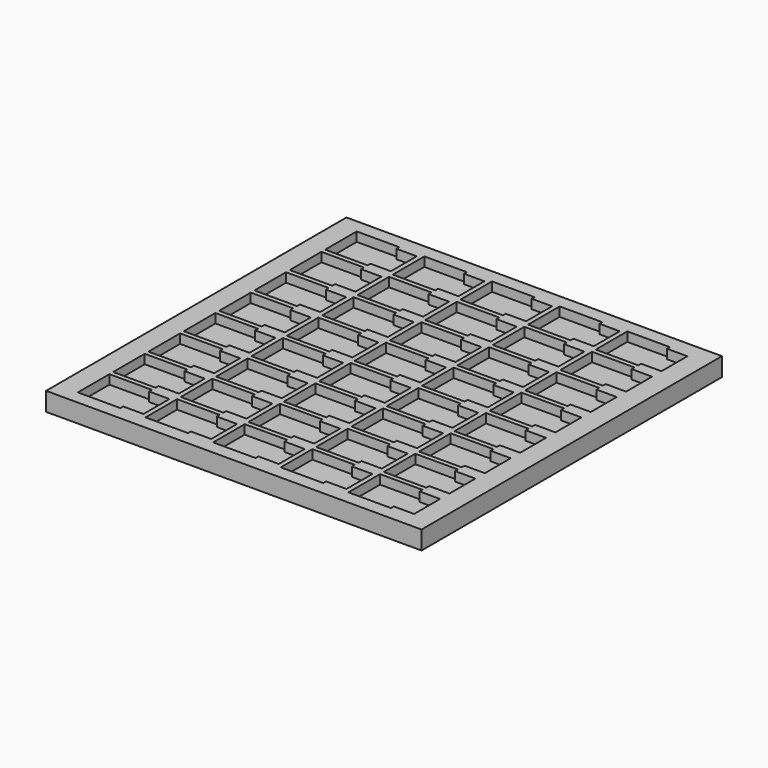
from build123d import *

# Parameters (mm, degrees)
F0_W     = 101.5
F0_H     = 101.5
F1_DEPTH = 5
F2_DEPTH = 2.5


# Not quite as in the source:
# - a feature names something its author has since deleted; it is built from what else it names


with BuildPart() as f1:
    # F0 (on Top) → F1 (new body)
    with BuildSketch(Plane.XY):
        Rectangle(F0_W, F0_H)
        Polygon((-33.5731, -46.1647), (-33.5731, -47.1182), (-45.0731, -47.1182), (-45.0731, -36.4482), (-33.5731, -36.4482), (-33.5731, -37.4017), (-28.0731, -37.4017), (-28.0731, -46.1647), align=None, mode=Mode.SUBTRACT)
        Polygon((-33.5731, -34.2267), (-33.5731, -35.1802), (-45.0731, -35.1802), (-45.0731, -24.5102), (-33.5731, -24.5102), (-33.5731, -25.4637), (-28.0731, -25.4637), (-28.0731, -34.2267), align=None, mode=Mode.SUBTRACT)
        Polygon((-15.2851, -46.1647), (-15.2851, -47.1182), (-26.7851, -47.1182), (-26.7851, -36.4482), (-15.2851, -36.4482), (-15.2851, -37.4017), (-9.7851, -37.4017), (-9.7851, -46.1647), align=None, mode=Mode.SUBTRACT)
        Polygon((-15.2851, -34.2267), (-15.2851, -35.1802), (-26.7851, -35.1802), (-26.7851, -24.5102), (-15.2851, -24.5102), (-15.2851, -25.4637), (-9.7851, -25.4637), (-9.7851, -34.2267), align=None, mode=Mode.SUBTRACT)
        Polygon((-33.5731, -22.2887), (-33.5731, -23.2422), (-45.0731, -23.2422), (-45.0731, -12.5722), (-33.5731, -12.5722), (-33.5731, -13.5257), (-28.0731, -13.5257), (-28.0731, -22.2887), align=None, mode=Mode.SUBTRACT)
        Polygon((-33.5731, -10.3507), (-33.5731, -11.3042), (-45.0731, -11.3042), (-45.0731, -0.6342), (-33.5731, -0.6342), (-33.5731, -1.5877), (-28.0731, -1.5877), (-28.0731, -10.3507), align=None, mode=Mode.SUBTRACT)
        Polygon((-15.2851, -22.2887), (-15.2851, -23.2422), (-26.7851, -23.2422), (-26.7851, -12.5722), (-15.2851, -12.5722), (-15.2851, -13.5257), (-9.7851, -13.5257), (-9.7851, -22.2887), align=None, mode=Mode.SUBTRACT)
        Polygon((-15.2851, -10.3507), (-15.2851, -11.3042), (-26.7851, -11.3042), (-26.7851, -0.6342), (-15.2851, -0.6342), (-15.2851, -1.5877), (-9.7851, -1.5877), (-9.7851, -10.3507), align=None, mode=Mode.SUBTRACT)
        Polygon((3.0029, -46.1647), (3.0029, -47.1182), (-8.4971, -47.1182), (-8.4971, -36.4482), (3.0029, -36.4482), (3.0029, -37.4017), (8.5029, -37.4017), (8.5029, -46.1647), align=None, mode=Mode.SUBTRACT)
        Polygon((21.2909, -46.1647), (21.2909, -47.1182), (9.7909, -47.1182), (9.7909, -36.4482), (21.2909, -36.4482), (21.2909, -37.4017), (26.7909, -37.4017), (26.7909, -46.1647), align=None, mode=Mode.SUBTRACT)
        Polygon((3.0029, -34.2267), (3.0029, -35.1802), (-8.4971, -35.1802), (-8.4971, -24.5102), (3.0029, -24.5102), (3.0029, -25.4637), (8.5029, -25.4637), (8.5029, -34.2267), align=None, mode=Mode.SUBTRACT)
        Polygon((21.2909, -34.2267), (21.2909, -35.1802), (9.7909, -35.1802), (9.7909, -24.5102), (21.2909, -24.5102), (21.2909, -25.4637), (26.7909, -25.4637), (26.7909, -34.2267), align=None, mode=Mode.SUBTRACT)
        Polygon((39.5789, -46.1647), (39.5789, -47.1182), (28.0789, -47.1182), (28.0789, -36.4482), (39.5789, -36.4482), (39.5789, -37.4017), (45.0789, -37.4017), (45.0789, -46.1647), align=None, mode=Mode.SUBTRACT)
        Polygon((39.5789, -34.2267), (39.5789, -35.1802), (28.0789, -35.1802), (28.0789, -24.5102), (39.5789, -24.5102), (39.5789, -25.4637), (45.0789, -25.4637), (45.0789, -34.2267), align=None, mode=Mode.SUBTRACT)
        Polygon((3.0029, -22.2887), (3.0029, -23.2422), (-8.4971, -23.2422), (-8.4971, -12.5722), (3.0029, -12.5722), (3.0029, -13.5257), (8.5029, -13.5257), (8.5029, -22.2887), align=None, mode=Mode.SUBTRACT)
        Polygon((21.2909, -22.2887), (21.2909, -23.2422), (9.7909, -23.2422), (9.7909, -12.5722), (21.2909, -12.5722), (21.2909, -13.5257), (26.7909, -13.5257), (26.7909, -22.2887), align=None, mode=Mode.SUBTRACT)
        Polygon((3.0029, -10.3507), (3.0029, -11.3042), (-8.4971, -11.3042), (-8.4971, -0.6342), (3.0029, -0.6342), (3.0029, -1.5877), (8.5029, -1.5877), (8.5029, -10.3507), align=None, mode=Mode.SUBTRACT)
        Polygon((21.2909, -10.3507), (21.2909, -11.3042), (9.7909, -11.3042), (9.7909, -0.6342), (21.2909, -0.6342), (21.2909, -1.5877), (26.7909, -1.5877), (26.7909, -10.3507), align=None, mode=Mode.SUBTRACT)
        Polygon((39.5789, -22.2887), (39.5789, -23.2422), (28.0789, -23.2422), (28.0789, -12.5722), (39.5789, -12.5722), (39.5789, -13.5257), (45.0789, -13.5257), (45.0789, -22.2887), align=None, mode=Mode.SUBTRACT)
        Polygon((39.5789, -10.3507), (39.5789, -11.3042), (28.0789, -11.3042), (28.0789, -0.6342), (39.5789, -0.6342), (39.5789, -1.5877), (45.0789, -1.5877), (45.0789, -10.3507), align=None, mode=Mode.SUBTRACT)
        Polygon((-33.5731, 1.5873), (-33.5731, 0.6338), (-45.0731, 0.6338), (-45.0731, 11.3038), (-33.5731, 11.3038), (-33.5731, 10.3503), (-28.0731, 10.3503), (-28.0731, 1.5873), align=None, mode=Mode.SUBTRACT)
        Polygon((-33.5731, 13.5253), (-33.5731, 12.5718), (-45.0731, 12.5718), (-45.0731, 23.2418), (-33.5731, 23.2418), (-33.5731, 22.2883), (-28.0731, 22.2883), (-28.0731, 13.5253), align=None, mode=Mode.SUBTRACT)
        Polygon((-15.2851, 1.5873), (-15.2851, 0.6338), (-26.7851, 0.6338), (-26.7851, 11.3038), (-15.2851, 11.3038), (-15.2851, 10.3503), (-9.7851, 10.3503), (-9.7851, 1.5873), align=None, mode=Mode.SUBTRACT)
        Polygon((-15.2851, 13.5253), (-15.2851, 12.5718), (-26.7851, 12.5718), (-26.7851, 23.2418), (-15.2851, 23.2418), (-15.2851, 22.2883), (-9.7851, 22.2883), (-9.7851, 13.5253), align=None, mode=Mode.SUBTRACT)
        Polygon((-33.5731, 25.4633), (-33.5731, 24.5098), (-45.0731, 24.5098), (-45.0731, 35.1798), (-33.5731, 35.1798), (-33.5731, 34.2263), (-28.0731, 34.2263), (-28.0731, 25.4633), align=None, mode=Mode.SUBTRACT)
        Polygon((-45.0731, 36.4478), (-45.0731, 47.1178), (-33.5731, 47.1178), (-33.5731, 46.1643), (-28.0731, 46.1643), (-28.0731, 37.4013), (-33.5731, 37.4013), (-33.5731, 36.4478), align=None, mode=Mode.SUBTRACT)
        Polygon((-15.2851, 25.4633), (-15.2851, 24.5098), (-26.7851, 24.5098), (-26.7851, 35.1798), (-15.2851, 35.1798), (-15.2851, 34.2263), (-9.7851, 34.2263), (-9.7851, 25.4633), align=None, mode=Mode.SUBTRACT)
        Polygon((-15.2851, 37.4013), (-15.2851, 36.4478), (-26.7851, 36.4478), (-26.7851, 47.1178), (-15.2851, 47.1178), (-15.2851, 46.1643), (-9.7851, 46.1643), (-9.7851, 37.4013), align=None, mode=Mode.SUBTRACT)
        Polygon((3.0029, 1.5873), (3.0029, 0.6338), (-8.4971, 0.6338), (-8.4971, 11.3038), (3.0029, 11.3038), (3.0029, 10.3503), (8.5029, 10.3503), (8.5029, 1.5873), align=None, mode=Mode.SUBTRACT)
        Polygon((21.2909, 1.5873), (21.2909, 0.6338), (9.7909, 0.6338), (9.7909, 11.3038), (21.2909, 11.3038), (21.2909, 10.3503), (26.7909, 10.3503), (26.7909, 1.5873), align=None, mode=Mode.SUBTRACT)
        Polygon((3.0029, 13.5253), (3.0029, 12.5718), (-8.4971, 12.5718), (-8.4971, 23.2418), (3.0029, 23.2418), (3.0029, 22.2883), (8.5029, 22.2883), (8.5029, 13.5253), align=None, mode=Mode.SUBTRACT)
        Polygon((21.2909, 13.5253), (21.2909, 12.5718), (9.7909, 12.5718), (9.7909, 23.2418), (21.2909, 23.2418), (21.2909, 22.2883), (26.7909, 22.2883), (26.7909, 13.5253), align=None, mode=Mode.SUBTRACT)
        Polygon((39.5789, 1.5873), (39.5789, 0.6338), (28.0789, 0.6338), (28.0789, 11.3038), (39.5789, 11.3038), (39.5789, 10.3503), (45.0789, 10.3503), (45.0789, 1.5873), align=None, mode=Mode.SUBTRACT)
        Polygon((39.5789, 13.5253), (39.5789, 12.5718), (28.0789, 12.5718), (28.0789, 23.2418), (39.5789, 23.2418), (39.5789, 22.2883), (45.0789, 22.2883), (45.0789, 13.5253), align=None, mode=Mode.SUBTRACT)
        Polygon((3.0029, 25.4633), (3.0029, 24.5098), (-8.4971, 24.5098), (-8.4971, 35.1798), (3.0029, 35.1798), (3.0029, 34.2263), (8.5029, 34.2263), (8.5029, 25.4633), align=None, mode=Mode.SUBTRACT)
        Polygon((21.2909, 25.4633), (21.2909, 24.5098), (9.7909, 24.5098), (9.7909, 35.1798), (21.2909, 35.1798), (21.2909, 34.2263), (26.7909, 34.2263), (26.7909, 25.4633), align=None, mode=Mode.SUBTRACT)
        Polygon((3.0029, 37.4013), (3.0029, 36.4478), (-8.4971, 36.4478), (-8.4971, 47.1178), (3.0029, 47.1178), (3.0029, 46.1643), (8.5029, 46.1643), (8.5029, 37.4013), align=None, mode=Mode.SUBTRACT)
        Polygon((21.2909, 37.4013), (21.2909, 36.4478), (9.7909, 36.4478), (9.7909, 47.1178), (21.2909, 47.1178), (21.2909, 46.1643), (26.7909, 46.1643), (26.7909, 37.4013), align=None, mode=Mode.SUBTRACT)
        Polygon((39.5789, 25.4633), (39.5789, 24.5098), (28.0789, 24.5098), (28.0789, 35.1798), (39.5789, 35.1798), (39.5789, 34.2263), (45.0789, 34.2263), (45.0789, 25.4633), align=None, mode=Mode.SUBTRACT)
        Polygon((39.5789, 37.4013), (39.5789, 36.4478), (28.0789, 36.4478), (28.0789, 47.1178), (39.5789, 47.1178), (39.5789, 46.1643), (45.0789, 46.1643), (45.0789, 37.4013), align=None, mode=Mode.SUBTRACT)
    extrude(amount=F1_DEPTH)

    # F0 (on Top) → F2 (join)
    with BuildSketch(Plane.XY):
        Polygon((-8.4971, -23.2422), (3.0029, -23.2422), (3.0029, -22.2887), (8.5029, -22.2887), (8.5029, -13.5257), (3.0029, -13.5257), (3.0029, -12.5722), (-8.4971, -12.5722), align=None)
        Polygon((28.0789, -11.3042), (39.5789, -11.3042), (39.5789, -10.3507), (45.0789, -10.3507), (45.0789, -1.5877), (39.5789, -1.5877), (39.5789, -0.6342), (28.0789, -0.6342), align=None)
        Polygon((-26.7851, 12.5718), (-15.2851, 12.5718), (-15.2851, 13.5253), (-9.7851, 13.5253), (-9.7851, 22.2883), (-15.2851, 22.2883), (-15.2851, 23.2418), (-26.7851, 23.2418), align=None)
        Polygon((9.7909, -35.1802), (21.2909, -35.1802), (21.2909, -34.2267), (26.7909, -34.2267), (26.7909, -25.4637), (21.2909, -25.4637), (21.2909, -24.5102), (9.7909, -24.5102), align=None)
        Polygon((-8.4971, 24.5098), (3.0029, 24.5098), (3.0029, 25.4633), (8.5029, 25.4633), (8.5029, 34.2263), (3.0029, 34.2263), (3.0029, 35.1798), (-8.4971, 35.1798), align=None)
        Polygon((-45.0731, -47.1182), (-33.5731, -47.1182), (-33.5731, -46.1647), (-28.0731, -46.1647), (-28.0731, -37.4017), (-33.5731, -37.4017), (-33.5731, -36.4482), (-45.0731, -36.4482), align=None)
        Polygon((-45.0731, 12.5718), (-33.5731, 12.5718), (-33.5731, 13.5253), (-28.0731, 13.5253), (-28.0731, 22.2883), (-33.5731, 22.2883), (-33.5731, 23.2418), (-45.0731, 23.2418), align=None)
        Polygon((28.0789, -23.2422), (39.5789, -23.2422), (39.5789, -22.2887), (45.0789, -22.2887), (45.0789, -13.5257), (39.5789, -13.5257), (39.5789, -12.5722), (28.0789, -12.5722), align=None)
        Polygon((9.7909, 24.5098), (21.2909, 24.5098), (21.2909, 25.4633), (26.7909, 25.4633), (26.7909, 34.2263), (21.2909, 34.2263), (21.2909, 35.1798), (9.7909, 35.1798), align=None)
        Polygon((28.0789, 24.5098), (39.5789, 24.5098), (39.5789, 25.4633), (45.0789, 25.4633), (45.0789, 34.2263), (39.5789, 34.2263), (39.5789, 35.1798), (28.0789, 35.1798), align=None)
        Polygon((28.0789, 0.6338), (39.5789, 0.6338), (39.5789, 1.5873), (45.0789, 1.5873), (45.0789, 10.3503), (39.5789, 10.3503), (39.5789, 11.3038), (28.0789, 11.3038), align=None)
        Polygon((-26.7851, -23.2422), (-15.2851, -23.2422), (-15.2851, -22.2887), (-9.7851, -22.2887), (-9.7851, -13.5257), (-15.2851, -13.5257), (-15.2851, -12.5722), (-26.7851, -12.5722), align=None)
        Polygon((-45.0731, -35.1802), (-33.5731, -35.1802), (-33.5731, -34.2267), (-28.0731, -34.2267), (-28.0731, -25.4637), (-33.5731, -25.4637), (-33.5731, -24.5102), (-45.0731, -24.5102), align=None)
        Polygon((-8.4971, -11.3042), (3.0029, -11.3042), (3.0029, -10.3507), (8.5029, -10.3507), (8.5029, -1.5877), (3.0029, -1.5877), (3.0029, -0.6342), (-8.4971, -0.6342), align=None)
        Polygon((-45.0731, -11.3042), (-33.5731, -11.3042), (-33.5731, -10.3507), (-28.0731, -10.3507), (-28.0731, -1.5877), (-33.5731, -1.5877), (-33.5731, -0.6342), (-45.0731, -0.6342), align=None)
        Polygon((-45.0731, 0.6338), (-33.5731, 0.6338), (-33.5731, 1.5873), (-28.0731, 1.5873), (-28.0731, 10.3503), (-33.5731, 10.3503), (-33.5731, 11.3038), (-45.0731, 11.3038), align=None)
        Polygon((-26.7851, -11.3042), (-15.2851, -11.3042), (-15.2851, -10.3507), (-9.7851, -10.3507), (-9.7851, -1.5877), (-15.2851, -1.5877), (-15.2851, -0.6342), (-26.7851, -0.6342), align=None)
        Polygon((28.0789, -35.1802), (39.5789, -35.1802), (39.5789, -34.2267), (45.0789, -34.2267), (45.0789, -25.4637), (39.5789, -25.4637), (39.5789, -24.5102), (28.0789, -24.5102), align=None)
        Polygon((9.7909, 12.5718), (21.2909, 12.5718), (21.2909, 13.5253), (26.7909, 13.5253), (26.7909, 22.2883), (21.2909, 22.2883), (21.2909, 23.2418), (9.7909, 23.2418), align=None)
        Polygon((-26.7851, -35.1802), (-15.2851, -35.1802), (-15.2851, -34.2267), (-9.7851, -34.2267), (-9.7851, -25.4637), (-15.2851, -25.4637), (-15.2851, -24.5102), (-26.7851, -24.5102), align=None)
        Polygon((9.7909, 36.4478), (21.2909, 36.4478), (21.2909, 37.4013), (26.7909, 37.4013), (26.7909, 46.1643), (21.2909, 46.1643), (21.2909, 47.1178), (9.7909, 47.1178), align=None)
        Polygon((-8.4971, -47.1182), (3.0029, -47.1182), (3.0029, -46.1647), (8.5029, -46.1647), (8.5029, -37.4017), (3.0029, -37.4017), (3.0029, -36.4482), (-8.4971, -36.4482), align=None)
        Polygon((9.7909, 0.6338), (21.2909, 0.6338), (21.2909, 1.5873), (26.7909, 1.5873), (26.7909, 10.3503), (21.2909, 10.3503), (21.2909, 11.3038), (9.7909, 11.3038), align=None)
        Polygon((-26.7851, -47.1182), (-15.2851, -47.1182), (-15.2851, -46.1647), (-9.7851, -46.1647), (-9.7851, -37.4017), (-15.2851, -37.4017), (-15.2851, -36.4482), (-26.7851, -36.4482), align=None)
        Polygon((-26.7851, 36.4478), (-15.2851, 36.4478), (-15.2851, 37.4013), (-9.7851, 37.4013), (-9.7851, 46.1643), (-15.2851, 46.1643), (-15.2851, 47.1178), (-26.7851, 47.1178), align=None)
        Polygon((-45.0731, -23.2422), (-33.5731, -23.2422), (-33.5731, -22.2887), (-28.0731, -22.2887), (-28.0731, -13.5257), (-33.5731, -13.5257), (-33.5731, -12.5722), (-45.0731, -12.5722), align=None)
        Polygon((28.0789, -47.1182), (39.5789, -47.1182), (39.5789, -46.1647), (45.0789, -46.1647), (45.0789, -37.4017), (39.5789, -37.4017), (39.5789, -36.4482), (28.0789, -36.4482), align=None)
        Polygon((28.0789, 36.4478), (39.5789, 36.4478), (39.5789, 37.4013), (45.0789, 37.4013), (45.0789, 46.1643), (39.5789, 46.1643), (39.5789, 47.1178), (28.0789, 47.1178), align=None)
        Polygon((-26.7851, 0.6338), (-15.2851, 0.6338), (-15.2851, 1.5873), (-9.7851, 1.5873), (-9.7851, 10.3503), (-15.2851, 10.3503), (-15.2851, 11.3038), (-26.7851, 11.3038), align=None)
        Polygon((-8.4971, 0.6338), (3.0029, 0.6338), (3.0029, 1.5873), (8.5029, 1.5873), (8.5029, 10.3503), (3.0029, 10.3503), (3.0029, 11.3038), (-8.4971, 11.3038), align=None)
        Polygon((-26.7851, 24.5098), (-15.2851, 24.5098), (-15.2851, 25.4633), (-9.7851, 25.4633), (-9.7851, 34.2263), (-15.2851, 34.2263), (-15.2851, 35.1798), (-26.7851, 35.1798), align=None)
        Polygon((28.0789, 12.5718), (39.5789, 12.5718), (39.5789, 13.5253), (45.0789, 13.5253), (45.0789, 22.2883), (39.5789, 22.2883), (39.5789, 23.2418), (28.0789, 23.2418), align=None)
        Polygon((9.7909, -11.3042), (21.2909, -11.3042), (21.2909, -10.3507), (26.7909, -10.3507), (26.7909, -1.5877), (21.2909, -1.5877), (21.2909, -0.6342), (9.7909, -0.6342), align=None)
        Polygon((-45.0731, 24.5098), (-33.5731, 24.5098), (-33.5731, 25.4633), (-28.0731, 25.4633), (-28.0731, 34.2263), (-33.5731, 34.2263), (-33.5731, 35.1798), (-45.0731, 35.1798), align=None)
        Polygon((-8.4971, 12.5718), (3.0029, 12.5718), (3.0029, 13.5253), (8.5029, 13.5253), (8.5029, 22.2883), (3.0029, 22.2883), (3.0029, 23.2418), (-8.4971, 23.2418), align=None)
        Polygon((9.7909, -47.1182), (21.2909, -47.1182), (21.2909, -46.1647), (26.7909, -46.1647), (26.7909, -37.4017), (21.2909, -37.4017), (21.2909, -36.4482), (9.7909, -36.4482), align=None)
        Polygon((-8.4971, -35.1802), (3.0029, -35.1802), (3.0029, -34.2267), (8.5029, -34.2267), (8.5029, -25.4637), (3.0029, -25.4637), (3.0029, -24.5102), (-8.4971, -24.5102), align=None)
        Polygon((-33.5731, 47.1178), (-45.0731, 47.1178), (-45.0731, 36.4478), (-33.5731, 36.4478), (-33.5731, 37.4013), (-28.0731, 37.4013), (-28.0731, 46.1643), (-33.5731, 46.1643), align=None)
        Polygon((-8.4971, 36.4478), (3.0029, 36.4478), (3.0029, 37.4013), (8.5029, 37.4013), (8.5029, 46.1643), (3.0029, 46.1643), (3.0029, 47.1178), (-8.4971, 47.1178), align=None)
        Polygon((9.7909, -23.2422), (21.2909, -23.2422), (21.2909, -22.2887), (26.7909, -22.2887), (26.7909, -13.5257), (21.2909, -13.5257), (21.2909, -12.5722), (9.7909, -12.5722), align=None)
    extrude(amount=F2_DEPTH)


solid = f1.part
